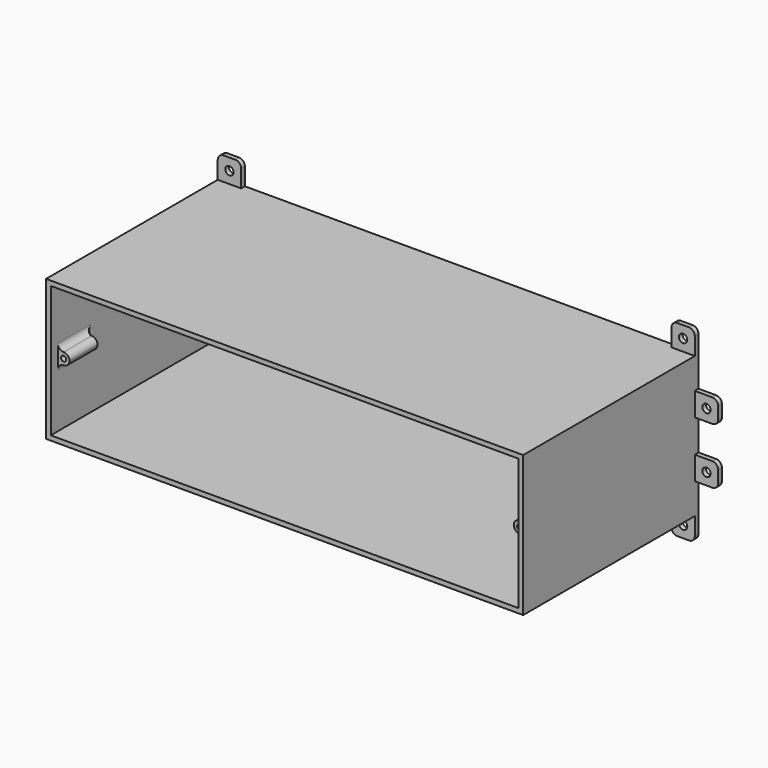
from build123d import *

# Parameters (mm, degrees)
F1_DEPTH     = 75
F0_W         = 8
F0_H         = 8
F0_R         = 1.425
F2_DEPTH     = 1.6
F3_R         = 2
F5_R         = 2
F6_START     = 60
F0_W_2       = 4
F0_H_2       = 4
F0_R_2       = 0.9
F6_DEPTH     = 12
F7_T1_DEPTH  = 12
F7_T6_DEPTH  = 4
F7_S7_R      = 0.9
F7_T8_DEPTH  = 4
F7_T13_DEPTH = 9
F7_T17_DEPTH = 17
F7_T24_DEPTH = 9
F7_T28_DEPTH = 17
F7_T31_DEPTH = 22
F9_R         = 2


# Not quite as in the source:
# - a fillet or chamfer that OpenCascade refuses, or shapes differently, is made with other operations: its cross-section is extruded or revolved along the edge and cut away or added


with BuildPart() as f1:
    # F0 (on Front) → F1 (new body)
    with BuildSketch(Plane.XZ):
        Polygon((-81.6, -13.6015841149), (-81.6, -24.1), (-73.6, -24.1), (73.6, -24.1), (81.6, -24.1), (81.6, -13.6015841149), (81.6, -5.6015841149), (81.6, 5.6015841149), (81.6, 13.6015841149), (81.6, 24.1), (73.6, 24.1), (-73.6, 24.1), (-81.6, 24.1), (-81.6, 13.6015841149), (-81.6, 5.6015841149), (-81.6, -5.6015841149), align=None)
        Polygon((80, -2), (80, -22.5), (-80, -22.5), (-80, 22.5), (80, 22.5), (80, 2), align=None, mode=Mode.SUBTRACT)
    extrude(amount=F1_DEPTH)

    # F0 (on Front) → F2 (join)
    with BuildSketch(Plane.XZ):
        Polygon((-81.6, -13.6015841149), (-81.6, -24.1), (-73.6, -24.1), (73.6, -24.1), (81.6, -24.1), (81.6, -13.6015841149), (81.6, -5.6015841149), (81.6, 5.6015841149), (81.6, 13.6015841149), (81.6, 24.1), (73.6, 24.1), (-73.6, 24.1), (-81.6, 24.1), (-81.6, 13.6015841149), (-81.6, 5.6015841149), (-81.6, -5.6015841149), align=None)
        Polygon((80, -2), (80, -22.5), (-80, -22.5), (-80, 22.5), (80, 22.5), (80, 2), align=None, mode=Mode.SUBTRACT)
        with Locations((-77.6, -28.1)):
            Rectangle(F0_W, F0_H)
        with Locations((-77.6, -28.1)):
            Circle(F0_R, mode=Mode.SUBTRACT)
        with Locations((-85.6, -9.6015841149)):
            Rectangle(F0_W, F0_H)
        with Locations((-85.6, -9.6015841149)):
            Circle(F0_R, mode=Mode.SUBTRACT)
        with Locations((77.6, -28.1)):
            Rectangle(F0_W, F0_H)
        with Locations((77.6, -28.1)):
            Circle(F0_R, mode=Mode.SUBTRACT)
        with Locations((-85.6, 9.6015841149)):
            Rectangle(F0_W, F0_H)
        with Locations((-85.6, 9.6015841149)):
            Circle(F0_R, mode=Mode.SUBTRACT)
        with Locations((85.6, -9.6015841149)):
            Rectangle(F0_W, F0_H)
        with Locations((85.6, -9.6015841149)):
            Circle(F0_R, mode=Mode.SUBTRACT)
        with Locations((-77.6, 28.1)):
            Rectangle(F0_W, F0_H)
        with Locations((-77.6, 28.1)):
            Circle(F0_R, mode=Mode.SUBTRACT)
        with Locations((85.6, 9.6015841149)):
            Rectangle(F0_W, F0_H)
        with Locations((85.6, 9.6015841149)):
            Circle(F0_R, mode=Mode.SUBTRACT)
        with Locations((77.6, 28.1)):
            Rectangle(F0_W, F0_H)
        with Locations((77.6, 28.1)):
            Circle(F0_R, mode=Mode.SUBTRACT)
    extrude(amount=F2_DEPTH)

    # F3
    f3_edges = [f1.edges().sort_by_distance(p)[0] for p in [
        (-81.6, -0.8, 32.1),
        (-73.6, -0.8, 32.1),
        (73.6, -0.8, 32.1),
        (81.6, -0.8, 32.1),
        (89.6, -0.8, -5.601584),
        (89.6, -0.8, -13.601584),
        (81.6, -0.8, -32.1),
        (73.6, -0.8, -32.1),
        (-89.6, -0.8, -13.601584),
        (-89.6, -0.8, -5.601584),
        (-81.6, -0.8, -32.1),
    ]]
    fillet(f3_edges, radius=F3_R)

    # F4: F1 across plane


with BuildPart() as f1_1:
    add(f1.part)
    add(f1.part.mirror(Plane.YZ))

    # F5
    f5_edges = [f1_1.edges().sort_by_distance(p)[0] for p in [
        (-73.6, -0.8, -32.1),
        (73.6, -0.8, -32.1),
    ]]
    fillet(f5_edges, radius=F5_R)

    # F0 (on Front) → F6 (join)
    with BuildSketch(Plane.XZ.offset(F6_START)):
        with Locations((78, 0)):
            Rectangle(F0_W_2, F0_H_2)
        with Locations((78, 0)):
            Circle(F0_R_2, mode=Mode.SUBTRACT)
    extrude(amount=F6_DEPTH)

    # F7: fillet of radius 2 on 5 edges, made by hand

    # F7_s2 → F7_t1 (join)
    with BuildSketch(Plane.XZ.offset(60)):
        with BuildLine():
            ThreePointArc((80, -4), (79.4142135624, -2.5857864376), (78, -2))
            Line((78, -2), (80, -2))
            Line((80, -2), (80, -4))
        make_face()
        with BuildLine():
            ThreePointArc((80, 4), (79.4142135624, 2.5857864376), (78, 2))
            Line((78, 2), (80, 2))
            Line((80, 2), (80, 4))
        make_face()
    extrude(amount=F7_T1_DEPTH)


with BuildPart() as f7_tool4:
    # F7_s5 → F7_t6 (new body)
    with BuildSketch(Plane.XY.offset(-2)):
        with BuildLine():
            ThreePointArc((80, -58), (79.4142135624, -59.4142135624), (78, -60))
            Line((78, -60), (80, -60))
            Line((80, -60), (80, -58))
        make_face()
    extrude(amount=F7_T6_DEPTH)

    # F7_s7 → F7_t8 (cut, symmetric)
    with BuildSketch(Plane.XZ.offset(59)):
        with Locations((78, 0)):
            Circle(F7_S7_R)
    extrude(amount=F7_T8_DEPTH, both=True, mode=Mode.SUBTRACT)


with BuildPart() as f1_2:
    add(f1_1.part)

    # F7_t3: union F7_tool4
    add(f7_tool4.part)


with BuildPart() as f7_tool11:
    # F7_s12 → F7_t13 (new body)
    with BuildSketch(Plane.XY.offset(-7)):
        with BuildLine():
            ThreePointArc((80, -58), (79.4142135624, -59.4142135624), (78, -60))
            Line((78, -60), (80, -60))
            Line((80, -60), (80, -58))
        make_face()
    extrude(amount=F7_T13_DEPTH)

    split(bisect_by=Plane.XY.offset(-2), keep=Keep.BOTTOM)


with BuildPart() as f7_tool15:
    # F7_s16 → F7_t17 (new body)
    with BuildSketch(Plane.XZ.offset(55)):
        with BuildLine():
            ThreePointArc((80, -4), (79.4142135624, -2.5857864376), (78, -2))
            Line((78, -2), (80, -2))
            Line((80, -2), (80, -4))
        make_face()
    extrude(amount=F7_T17_DEPTH)

    split(bisect_by=Plane.XZ.offset(60), keep=Keep.BOTTOM)


with BuildPart() as f7_tool11_1:
    add(f7_tool11.part)

    # F7_t19: intersect F7_tool15
    add(f7_tool15.part, mode=Mode.INTERSECT)


with BuildPart() as f1_3:
    add(f1_2.part)

    # F7_t9: union F7_tool11
    add(f7_tool11_1.part)


with BuildPart() as f7_tool22:
    # F7_s23 → F7_t24 (new body)
    with BuildSketch(Plane.XY.offset(-2)):
        with BuildLine():
            ThreePointArc((80, -58), (79.4142135624, -59.4142135624), (78, -60))
            Line((78, -60), (80, -60))
            Line((80, -60), (80, -58))
        make_face()
    extrude(amount=F7_T24_DEPTH)

    split(bisect_by=Plane.XY.offset(2), keep=Keep.TOP)


with BuildPart() as f7_tool26:
    # F7_s27 → F7_t28 (new body)
    with BuildSketch(Plane.XZ.offset(55)):
        with BuildLine():
            ThreePointArc((80, 4), (79.4142135624, 2.5857864376), (78, 2))
            Line((78, 2), (80, 2))
            Line((80, 2), (80, 4))
        make_face()
    extrude(amount=F7_T28_DEPTH)

    split(bisect_by=Plane.XZ.offset(60), keep=Keep.BOTTOM)


with BuildPart() as f7_tool22_1:
    add(f7_tool22.part)

    # F7_t30: intersect F7_tool26
    add(f7_tool26.part, mode=Mode.INTERSECT)


with BuildPart() as f1_4:
    add(f1_3.part)

    # F7_t20: union F7_tool22
    add(f7_tool22_1.part)

    # F7_s32 → F7_t31 (cut)
    with BuildSketch(Plane.XZ.offset(55)):
        with BuildLine():
            ThreePointArc((78, -2), (76.5857864376, -1.4142135624), (76, 0))
            Line((76, 0), (76, -2))
            Line((76, -2), (78, -2))
        make_face()
        with BuildLine():
            ThreePointArc((78, 2), (76.5857864376, 1.4142135624), (76, 0))
            Line((76, 0), (76, 2))
            Line((76, 2), (78, 2))
        make_face()
    extrude(amount=F7_T31_DEPTH, mode=Mode.SUBTRACT)

    # F8: F1 across plane


with BuildPart() as f1_5:
    add(f1_4.part)
    add(f1_4.part.mirror(Plane.YZ))

    # F9
    f9_edges = [f1_5.edges().sort_by_distance(p)[0] for p in [
        (89.6, -0.8, 5.601584),
        (89.6, -0.8, 13.601584),
        (-89.6, -0.8, 5.601584),
        (-89.6, -0.8, 13.601584),
    ]]
    fillet(f9_edges, radius=F9_R)


solid = f1_5.part
